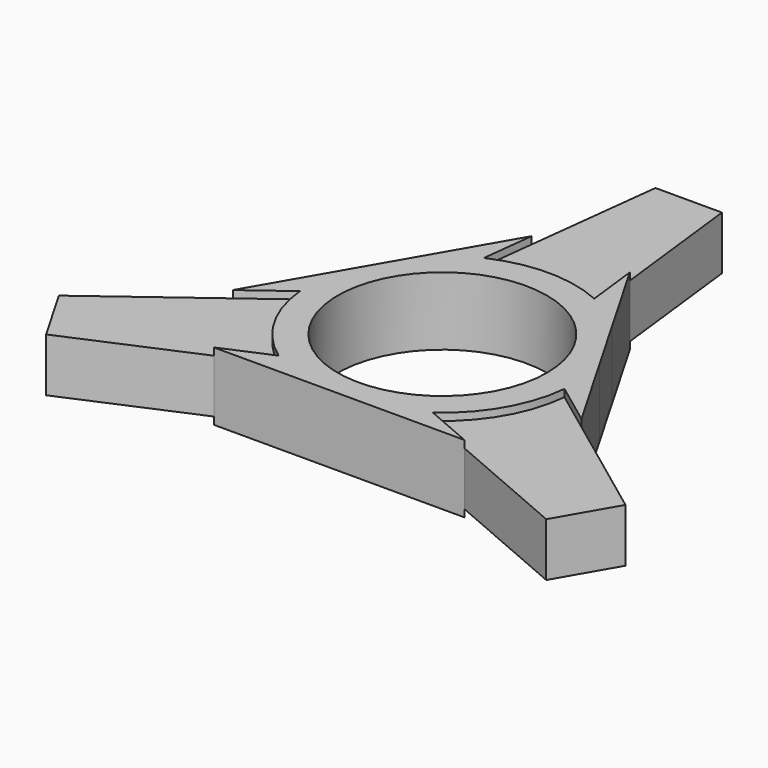
from build123d import *

# Parameters (mm, degrees)
F0_R     = 10.922
F1_DEPTH = 7.112
F2_DEPTH = 6.35
F3_DEPTH = 0.762
F4_DEPTH = 7.112


with BuildPart() as f1:
    # F0 (on Top) → F1 (new body)
    with BuildSketch(Plane.XY):
        with BuildLine():
            Line((-5.7560840378, 12.6157379826), (-5.1183423957, 18.0540294813))
            Line((-5.1183423957, 18.0540294813), (-9.9884684203, 9.6187237673))
            ThreePointArc((-9.9884684203, 9.6187237673), (-8.0136294261, 11.3168499026), (-5.7560840378, 12.6157379826))
        make_face()
        with BuildLine():
            ThreePointArc((5.7560840378, 12.6157379826), (0, 13.8668434871), (-5.7560840378, 12.6157379826))
            ThreePointArc((-5.7560840378, 12.6157379826), (-8.0136294261, 11.3168499026), (-9.9884684203, 9.6187237673))
            Line((-9.9884684203, 9.6187237673), (-13.3242933447, 3.8409055132))
            ThreePointArc((-13.3242933447, 3.8409055132), (-13.8074942195, 1.2815817082), (-13.8035915993, -1.3229539883))
            ThreePointArc((-13.8035915993, -1.3229539883), (-12.0090387301, -6.9334217436), (-8.0475075615, -11.2927839943))
            ThreePointArc((-8.0475075615, -11.2927839943), (-5.7938647934, -12.5984316108), (-3.3358249243, -13.4596292806))
            Line((-3.3358249243, -13.4596292806), (3.3358249243, -13.4596292806))
            ThreePointArc((3.3358249243, -13.4596292806), (5.7938647934, -12.5984316108), (8.0475075615, -11.2927839943))
            ThreePointArc((8.0475075615, -11.2927839943), (12.0090387301, -6.9334217436), (13.8035915993, -1.3229539883))
            ThreePointArc((13.8035915993, -1.3229539883), (13.8510214888, -0.6622325982), (13.8668434871, 0))
            ThreePointArc((13.8668434871, 0), (13.730536018, 1.9395177119), (13.3242933447, 3.8409055132))
            Line((13.3242933447, 3.8409055132), (9.9884684203, 9.6187237673))
            ThreePointArc((9.9884684203, 9.6187237673), (8.0136294261, 11.3168499026), (5.7560840378, 12.6157379826))
        make_face()
        Circle(F0_R, mode=Mode.SUBTRACT)
        with BuildLine():
            Line((5.1183423957, 18.0540294813), (5.7560840378, 12.6157379826))
            ThreePointArc((5.7560840378, 12.6157379826), (8.0136294261, 11.3168499026), (9.9884684203, 9.6187237673))
            Line((9.9884684203, 9.6187237673), (5.1183423957, 18.0540294813))
        make_face()
        with BuildLine():
            ThreePointArc((-13.8035915993, -1.3229539883), (-13.8074942195, 1.2815817082), (-13.3242933447, 3.8409055132))
            Line((-13.3242933447, 3.8409055132), (-18.1944193693, -4.5944002008))
            Line((-18.1944193693, -4.5944002008), (-13.8035915993, -1.3229539883))
        make_face()
        with BuildLine():
            Line((18.1944193693, -4.5944002008), (13.3242933447, 3.8409055132))
            ThreePointArc((13.3242933447, 3.8409055132), (13.730536018, 1.9395177119), (13.8668434871, 0))
            ThreePointArc((13.8668434871, 0), (13.8510214888, -0.6622325982), (13.8035915993, -1.3229539883))
            Line((13.8035915993, -1.3229539883), (18.1944193693, -4.5944002008))
        make_face()
        with BuildLine():
            ThreePointArc((8.0475075615, -11.2927839943), (5.7938647934, -12.5984316108), (3.3358249243, -13.4596292806))
            Line((3.3358249243, -13.4596292806), (13.0760769737, -13.4596292806))
            Line((13.0760769737, -13.4596292806), (8.0475075615, -11.2927839943))
        make_face()
    extrude(amount=F1_DEPTH)

    # F0 (on Top) → F2 (join)
    with BuildSketch(Plane.XY):
        with BuildLine():
            ThreePointArc((-8.0475075615, -11.2927839943), (-12.0090387301, -6.9334217436), (-13.8035915993, -1.3229539883))
            Line((-13.8035915993, -1.3229539883), (-18.1944193693, -4.5944002008))
            Line((-18.1944193693, -4.5944002008), (-29.5624734591, -13.0643241977))
            Line((-29.5624734591, -13.0643241977), (-26.095273368, -19.0696909155))
            Line((-26.095273368, -19.0696909155), (-13.0760769737, -13.4596292806))
            Line((-13.0760769737, -13.4596292806), (-8.0475075615, -11.2927839943))
        make_face()
        with BuildLine():
            Line((-3.4672000911, 32.1340151131), (-5.1183423957, 18.0540294813))
            Line((-5.1183423957, 18.0540294813), (-5.7560840378, 12.6157379826))
            ThreePointArc((-5.7560840378, 12.6157379826), (0, 13.8668434871), (5.7560840378, 12.6157379826))
            Line((5.7560840378, 12.6157379826), (5.1183423957, 18.0540294813))
            Line((5.1183423957, 18.0540294813), (3.4672000911, 32.1340151131))
            Line((3.4672000911, 32.1340151131), (-3.4672000911, 32.1340151131))
        make_face()
        with BuildLine():
            Line((29.5624734591, -13.0643241977), (18.1944193693, -4.5944002008))
            Line((18.1944193693, -4.5944002008), (13.8035915993, -1.3229539883))
            ThreePointArc((13.8035915993, -1.3229539883), (12.0090387301, -6.9334217436), (8.0475075615, -11.2927839943))
            Line((8.0475075615, -11.2927839943), (13.0760769737, -13.4596292806))
            Line((13.0760769737, -13.4596292806), (26.095273368, -19.0696909155))
            Line((26.095273368, -19.0696909155), (29.5624734591, -13.0643241977))
        make_face()
    extrude(amount=F2_DEPTH)

    # F0 (on Top) → F3 (cut)
    with BuildSketch(Plane.XY):
        with BuildLine():
            Line((29.5624734591, -13.0643241977), (18.1944193693, -4.5944002008))
            Line((18.1944193693, -4.5944002008), (13.8035915993, -1.3229539883))
            ThreePointArc((13.8035915993, -1.3229539883), (12.0090387301, -6.9334217436), (8.0475075615, -11.2927839943))
            Line((8.0475075615, -11.2927839943), (13.0760769737, -13.4596292806))
            Line((13.0760769737, -13.4596292806), (26.095273368, -19.0696909155))
            Line((26.095273368, -19.0696909155), (29.5624734591, -13.0643241977))
        make_face()
        with BuildLine():
            Line((-3.4672000911, 32.1340151131), (-5.1183423957, 18.0540294813))
            Line((-5.1183423957, 18.0540294813), (-5.7560840378, 12.6157379826))
            ThreePointArc((-5.7560840378, 12.6157379826), (0, 13.8668434871), (5.7560840378, 12.6157379826))
            Line((5.7560840378, 12.6157379826), (5.1183423957, 18.0540294813))
            Line((5.1183423957, 18.0540294813), (3.4672000911, 32.1340151131))
            Line((3.4672000911, 32.1340151131), (-3.4672000911, 32.1340151131))
        make_face()
        with BuildLine():
            ThreePointArc((-8.0475075615, -11.2927839943), (-12.0090387301, -6.9334217436), (-13.8035915993, -1.3229539883))
            Line((-13.8035915993, -1.3229539883), (-18.1944193693, -4.5944002008))
            Line((-18.1944193693, -4.5944002008), (-29.5624734591, -13.0643241977))
            Line((-29.5624734591, -13.0643241977), (-26.095273368, -19.0696909155))
            Line((-26.095273368, -19.0696909155), (-13.0760769737, -13.4596292806))
            Line((-13.0760769737, -13.4596292806), (-8.0475075615, -11.2927839943))
        make_face()
    extrude(amount=F3_DEPTH, mode=Mode.SUBTRACT)

    # F0 (on Top) → F4 (join)
    with BuildSketch(Plane.XY):
        with BuildLine():
            ThreePointArc((-3.3358249243, -13.4596292806), (-5.7938647934, -12.5984316108), (-8.0475075615, -11.2927839943))
            Line((-8.0475075615, -11.2927839943), (-13.0760769737, -13.4596292806))
            Line((-13.0760769737, -13.4596292806), (-3.3358249243, -13.4596292806))
        make_face()
    extrude(amount=F4_DEPTH)


solid = f1.part
